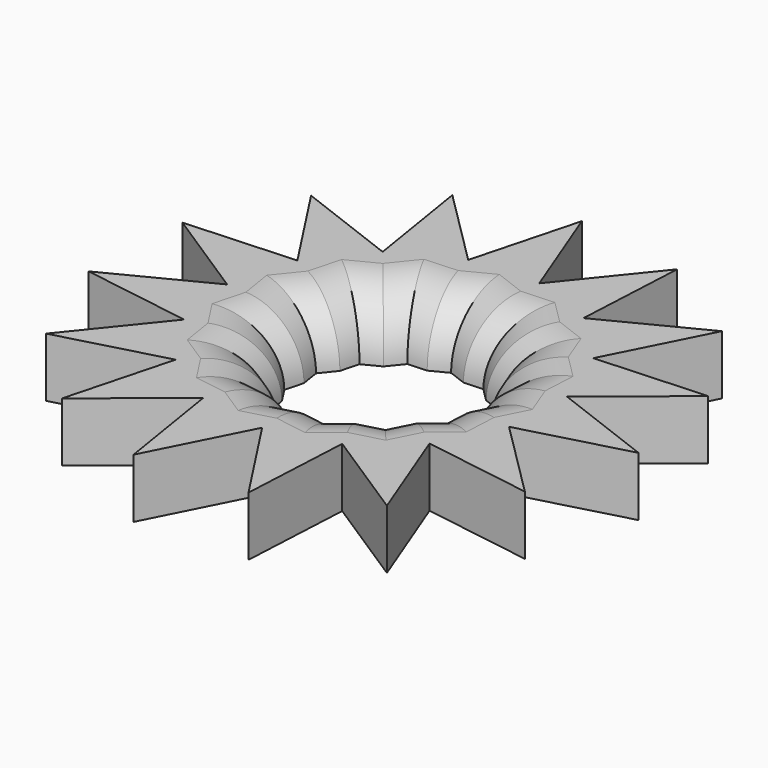
from build123d import *

# Parameters (mm, degrees)
F1_DEPTH = 5.08
F2_R     = 5.07999


# Not quite as in the source:
# - a fillet or chamfer is up to 0.001 mm smaller than in the source, because OpenCascade refuses the exact size


with BuildPart() as f1:
    # F0 (on Top) → F1 (new body)
    with BuildSketch(Plane.XY):
        Polygon((-21.999723834, 5.8521262697), (-14.0514369357, 0.7108895722), (-10.1598827967, 2.7026210629), (-12.5474815477, 6.3646642291), align=None)
        Polygon((-22.4780219717, -3.6019104497), (-13.1257712241, -5.0658043501), (-10.3807697977, -1.6634294271), (-14.0514369357, 0.7108895722), align=None)
        Polygon((-19.0696659041, -12.4331441299), (-9.930540424, -9.9665746788), (-8.8067273944, -5.7418578572), (-13.1257712241, -5.0658043501), align=None)
        Polygon((-9.930540424, -9.9665746788), (-12.3639913592, -19.1145742385), (-5.0182289685, -13.144033702), (-5.7099218179, -8.8274669008), align=None)
        Polygon((-1.6258188862, -10.3867267222), (-5.0182289685, -13.144033702), (-3.5204703849, -22.4909208108), (0.7617798649, -14.0487698884), align=None)
        Polygon((2.7394029011, -10.1500271328), (0.7617798649, -14.0487698884), (5.9317719013, -21.9783828513), (6.4100700391, -12.524346132), align=None)
        Polygon((6.6309570401, -8.1582956421), (6.4100700391, -12.524346132), (14.3583569374, -17.6655828295), (10.9500008698, -8.8343491493), align=None)
        Polygon((9.3759584665, -4.7559207191), (10.9500008698, -8.8343491493), (20.3022516175, -10.2982430497), (13.5965770725, -3.6168129411), align=None)
        Polygon((10.4997714961, -0.5312038976), (13.5965770725, -3.6168129411), (22.7357025527, -1.15024349), (13.8921815784, 2.2261030823), align=None)
        Polygon((9.8080786466, 3.7853629037), (13.8921815784, 2.2261030823), (21.2379439691, 8.1966436188), (11.7857016829, 7.6841056593), align=None)
        Polygon((7.6413668966, 11.8134565599), (7.4204798956, 7.44740607), (11.7857016829, 7.6841056593), (16.0679519327, 16.1262565817), align=None)
        Polygon((8.1196650343, 21.2674932792), (2.1757703543, 13.9001534994), (3.7498127576, 9.8217250692), (7.6413668966, 11.8134565599), align=None)
        Polygon((-1.2325857133, 22.7313871796), (-3.6660366485, 13.5833876199), (-0.5692310721, 10.4977785763), (2.1757703543, 13.9001534994), align=None)
        Polygon((-8.8739526099, 10.9179306197), (-4.7898496782, 9.3586707984), (-3.6660366485, 13.5833876199), (-10.3717111935, 20.2648177285), align=None)
        Polygon((-17.7174735842, 14.294277192), (-12.5474815477, 6.3646642291), (-8.1822597605, 6.6013638185), (-8.8739526099, 10.9179306197), align=None)
        Polygon((-12.5474815477, 6.3646642291), (-10.1598827967, 2.7026210629), (-7.7547700697, 3.9335788206), (-8.1822597605, 6.6013638185), align=None)
        Polygon((-14.0514369357, 0.7108895722), (-10.3807697977, -1.6634294271), (-8.684265617, 0.4393539178), (-10.1598827967, 2.7026210629), align=None)
        Polygon((-13.1257712241, -5.0658043501), (-8.8067273944, -5.7418578572), (-8.112172745, -3.1308392687), (-10.3807697977, -1.6634294271), align=None)
        Polygon((-8.8067273944, -5.7418578572), (-9.930540424, -9.9665746788), (-5.7099218179, -8.8274669008), (-6.1374115087, -6.1596819029), align=None)
        Polygon((-5.7099218179, -8.8274669008), (-5.0182289685, -13.144033702), (-1.6258188862, -10.3867267222), (-3.1014360658, -8.1234595771), align=None)
        Polygon((0.4708058484, -8.6826172912), (-1.6258188862, -10.3867267222), (0.7617798649, -14.0487698884), (2.7394029011, -10.1500271328), align=None)
        Polygon((3.9616411544, -7.7404715965), (2.7394029011, -10.1500271328), (6.4100700391, -12.524346132), (6.6309570401, -8.1582956421), align=None)
        Polygon((6.7674727144, -5.4599280427), (6.6309570401, -8.1582956421), (10.9500008698, -8.8343491493), (9.3759584665, -4.7559207191), align=None)
        Polygon((8.4031467615, -2.2353133286), (9.3759584665, -4.7559207191), (13.5965770725, -3.6168129411), (10.4997714961, -0.5312038976), align=None)
        Polygon((8.5858403933, 1.3758073673), (10.4997714961, -0.5312038976), (13.8921815784, 2.2261030823), (9.8080786466, 3.7853629037), align=None)
        Polygon((7.4204798956, 7.44740607), (7.2839642213, 4.7490384706), (9.8080786466, 3.7853629037), (11.7857016829, 7.6841056593), align=None)
        Polygon((3.7498127576, 9.8217250692), (4.7226244626, 7.3011176786), (7.4204798956, 7.44740607), (7.6413668966, 11.8134565599), align=None)
        Polygon((2.1757703543, 13.9001534994), (-0.5692310721, 10.4977785763), (1.3447000307, 8.5907673114), (3.7498127576, 9.8217250692), align=None)
        Polygon((-3.6660366485, 13.5833876199), (-4.7898496782, 9.3586707984), (-2.2657352528, 8.3949952315), (-0.5692310721, 10.4977785763), align=None)
        Polygon((-8.1822597605, 6.6013638185), (-5.4844043275, 6.7476522098), (-4.7898496782, 9.3586707984), (-8.8739526099, 10.9179306197), align=None)
        Polygon((-10.1598827967, 2.7026210629), (-8.684265617, 0.4393539178), (-7.4416532636, 1.979547329), (-7.7547700697, 3.9335788206), align=None)
        Polygon((-10.3807697977, -1.6634294271), (-8.112172745, -3.1308392687), (-7.6034429717, -1.2183865968), (-8.684265617, 0.4393539178), align=None)
        Polygon((-8.112172745, -3.1308392687), (-8.8067273944, -5.7418578572), (-6.1374115087, -6.1596819029), (-6.4505283149, -4.2056504113), align=None)
        Polygon((-6.1374115087, -6.1596819029), (-5.7099218179, -8.8274669008), (-3.1014360658, -8.1234595771), (-4.1822587112, -6.4657190625), align=None)
        Polygon((-3.1014360658, -8.1234595771), (-1.6258188862, -10.3867267222), (0.4708058484, -8.6826172912), (-1.1908385817, -7.6078061486), align=None)
        Polygon((2.0064883569, -7.4344344369), (0.4708058484, -8.6826172912), (2.7394029011, -10.1500271328), (3.9616411544, -7.7404715965), align=None)
        Polygon((4.8568752303, -5.9755814713), (3.9616411544, -7.7404715965), (6.6309570401, -8.1582956421), (6.7674727144, -5.4599280427), align=None)
        Polygon((6.867464253, -3.4834961829), (6.7674727144, -5.4599280427), (9.3759584665, -4.7559207191), (8.4031467615, -2.2353133286), align=None)
        Polygon((7.6906063175, -0.3890827578), (8.4031467615, -2.2353133286), (10.4997714961, -0.5312038976), (8.5858403933, 1.3758073673), align=None)
        Polygon((7.2839642213, 4.7490384706), (7.1839726826, 2.7726066107), (8.5858403933, 1.3758073673), (9.8080786466, 3.7853629037), align=None)
        Polygon((4.7226244626, 7.3011176786), (5.4351649066, 5.4548871079), (7.2839642213, 4.7490384706), (7.4204798956, 7.44740607), align=None)
        Polygon((-0.5692310721, 10.4977785763), (-2.2657352528, 8.3949952315), (-0.4169359382, 7.6891465941), (1.3447000307, 8.5907673114), align=None)
        Polygon((-4.7898496782, 9.3586707984), (-5.4844043275, 6.7476522098), (-3.5083476063, 6.8548018203), (-2.2657352528, 8.3949952315), align=None)
        Polygon((-7.4416532636, 1.979547329), (-6.4138998748, 3.2534273071), (-5.9931341009, 4.8351995379), (-7.7547700697, 3.9335788206), align=None)
        Polygon((-8.684265617, 0.4393539178), (-7.6034429717, -1.2183865968), (-7.1826771978, 0.363385634), (-7.4416532636, 1.979547329), align=None)
        Polygon((-7.6034429717, -1.2183865968), (-8.112172745, -3.1308392687), (-6.4505283149, -4.2056504113), (-6.7095043807, -2.5894887164), align=None)
        Polygon((-6.4505283149, -4.2056504113), (-6.1374115087, -6.1596819029), (-4.1822587112, -6.4657190625), (-5.0761973022, -5.0946169429), align=None)
        Polygon((-4.1822587112, -6.4657190625), (-3.1014360658, -8.1234595771), (-1.1908385817, -7.6078061486), (-2.5651695944, -6.7188396169), align=None)
        Polygon((-1.1908385817, -7.6078061486), (0.4708058484, -8.6826172912), (2.0064883569, -7.4344344369), (0.3893992401, -7.1813138824), align=None)
        Polygon((3.2766374084, -6.4020737375), (2.0064883569, -7.4344344369), (3.9616411544, -7.7404715965), (4.8568752303, -5.9755814713), align=None)
        Polygon((5.5973152015, -4.5158568823), (4.8568752303, -5.9755814713), (6.7674727144, -5.4599280427), (6.867464253, -3.4834961829), align=None)
        Polygon((6.9501663462, -1.8488073469), (6.867464253, -3.4834961829), (8.4031467615, -2.2353133286), (7.6906063175, -0.3890827578), align=None)
        Polygon((7.1839726826, 2.7726066107), (7.1012705894, 1.1379177747), (7.6906063175, -0.3890827578), (8.5858403933, 1.3758073673), align=None)
        Polygon((1.3447000307, 8.5907673114), (2.7465677414, 7.1939680681), (4.7226244626, 7.3011176786), (3.7498127576, 9.8217250692), align=None)
        Polygon((4.7226244626, 7.3011176786), (2.7465677414, 7.1939680681), (3.9060397893, 6.0386881034), (5.4351649066, 5.4548871079), align=None)
        Polygon((-0.4169359382, 7.6891465941), (1.1121891791, 7.1053455986), (2.7465677414, 7.1939680681), (1.3447000307, 8.5907673114), align=None)
        Polygon((-2.2657352528, 8.3949952315), (-3.5083476063, 6.8548018203), (-1.873969044, 6.9434242898), (-0.4169359382, 7.6891465941), align=None)
        Polygon((-5.4844043275, 6.7476522098), (-5.9931341009, 4.8351995379), (-4.536100995, 5.5809218422), (-3.5083476063, 6.8548018203), align=None)
        Polygon((-7.7547700697, 3.9335788206), (-5.9931341009, 4.8351995379), (-5.4844043275, 6.7476522098), (-8.1822597605, 6.6013638185), align=None)
        Polygon((5.4351649066, 5.4548871079), (6.0245006347, 3.9278865754), (7.1839726826, 2.7726066107), (7.2839642213, 4.7490384706), align=None)
    extrude(amount=F1_DEPTH)

    # F2 (radius 5.08 in the source; OpenCascade refuses exactly that, so slightly less here)
    f2_edges = [f1.edges().sort_by_distance(p)[0] for p in [
        (-6.203517, 4.044313, 5.08),
        (-6.927777, 2.616487, 5.08),
        (-7.312165, 1.171466, 5.08),
        (-7.39306, -0.4275, 5.08),
        (-7.156474, -1.903938, 5.08),
        (-6.580016, -3.39757, 5.08),
        (-5.763363, -4.650134, 5.08),
        (-4.629228, -5.780168, 5.08),
        (-3.373714, -6.592279, 5.08),
        (-1.878004, -7.163323, 5.08),
        (-0.40072, -7.39456, 5.08),
        (1.197944, -7.307874, 5.08),
        (2.641563, -6.918254, 5.08),
        (4.066756, -6.188828, 5.08),
        (5.227095, -5.245719, 5.08),
        (6.908815, -2.666152, 5.08),
        (7.320386, -1.118945, 5.08),
        (7.395938, 0.374418, 5.08),
        (7.142622, 1.955262, 5.08),
        (6.604237, 3.350247, 5.08),
        (3.326304, 6.616328, 5.08),
        (5.729833, 4.691387, 5.08),
        (4.670602, 5.746788, 5.08),
        (1.929378, 7.149657, 5.08),
        (0.347627, 7.397246, 5.08),
        (-1.145452, 7.316285, 5.08),
        (-2.691158, 6.899113, 5.08),
        (-4.022224, 6.217862, 5.08),
        (-5.264618, 5.208061, 5.08),
        (6.23239, -3.999677, 5.08),
    ]]
    fillet(f2_edges, radius=F2_R)


solid = f1.part
